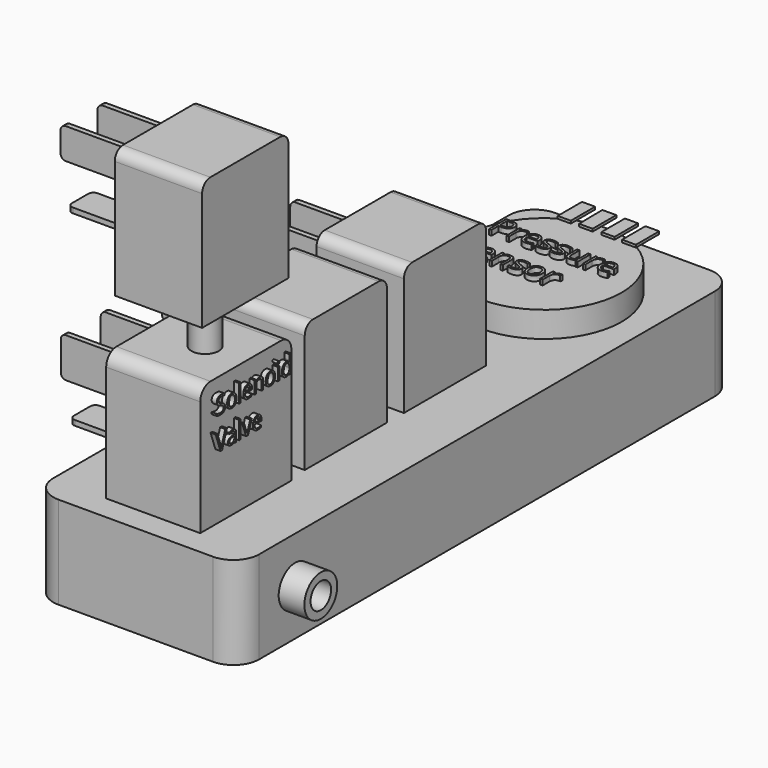
from build123d import *

# Parameters (mm, degrees)
F0_W          = 40.0781370699
F0_H          = 120.8194904029
F1_DEPTH      = 18
F2_R          = 15.0946600393
F3_DEPTH      = 5
F5_DEPTH      = 0.5
F7_DEPTH      = 0.5
F9_DEPTH      = 0.5
F10_TEXT_SIZE = 5.8368311741
F11_DEPTH     = 1
F12_R         = 4
F13_DEPTH     = 5
F15_D         = 5
F15_DEPTH     = 10
F15_TIP       = 1.5021515476
F17_DEPTH     = 0.5
F18_R         = 4
F19_DEPTH     = 5
F21_D         = 5
F21_DEPTH     = 10
F21_TIP       = 1.5021515476
F22_R         = 5
F23_R         = 5
F24_R         = 5
F25_R         = 5
F26_W         = 18.3048888575
F26_H         = 22.1605543047
F27_DEPTH     = 25
F28_R         = 2.5
F29_TEXT_SIZE = 4.6175733077
F30_DEPTH     = 1
F31_W         = 17
F31_H         = 20
F32_DEPTH     = 25
F33_R         = 2
F35_W         = 1
F35_H         = 7.7205877751
F35_W_2       = 6
F35_H_2       = 1
F36_DEPTH     = 15
F37_R         = 2.6676591168
F38_DEPTH     = 10
F39_W         = 17
F39_H         = 21
F40_DEPTH     = 25
F41_R         = 2
F42_W         = 1
F42_H         = 6
F42_W_2       = 6
F42_H_2       = 1
F43_DEPTH     = 15
F44_R         = 1


# Not quite as in the source:
# - Text() gives the source's letters only with a copy of the font that has no kerning and outlines rounded to 1/6400 em; it was checked with that copy


with BuildPart() as f1:
    # F0 (on Top) → F1 (new body)
    with BuildSketch(Plane.XY):
        with Locations((-11.1165624112, 8.9225042611)):
            Rectangle(F0_W, F0_H)
    extrude(amount=F1_DEPTH)

    # F2 (on face) → F3 (join)
    with BuildSketch(Plane.XY.offset(18)):
        with Locations((-10.9592955559, 47.6713515818)):
            Circle(F2_R)
    extrude(amount=F3_DEPTH)

    # F4 (on face) → F5 (join)
    with BuildSketch(Plane.XY.offset(23)):
        with BuildLine():
            Line((-14.5544850931, 66.3335174322), (-14.4999837088, 62.3448749864))
            ThreePointArc((-14.4999837088, 62.3448749864), (-13.1815212085, 62.6015382803), (-11.8454620242, 62.7399769568))
            Line((-11.8454620242, 62.7399769568), (-11.8454620242, 66.3335174322))
            Line((-11.8454620242, 66.3335174322), (-14.5544850931, 66.3335174322))
        make_face()
        with BuildLine():
            Line((-14.4999837088, 62.3448749864), (-14.4758609787, 60.5794712901))
            Line((-14.4758609787, 60.5794712901), (-11.8454620242, 60.5794712901))
            Line((-11.8454620242, 60.5794712901), (-11.8454620242, 62.7399769568))
            ThreePointArc((-11.8454620242, 62.7399769568), (-13.1815212085, 62.6015382803), (-14.4999837088, 62.3448749864))
        make_face()
    extrude(amount=F5_DEPTH)

    # F6 (on face) → F7 (join)
    with BuildSketch(Plane.XY.offset(23)):
        with BuildLine():
            Line((-18.6310531572, 60.5794712901), (-16.0875776783, 60.5794712901))
            Line((-16.0875776783, 60.5794712901), (-16.0875776783, 61.8681640471))
            ThreePointArc((-16.0875776783, 61.8681640471), (-17.3872429539, 61.3289594965), (-18.6310531572, 60.671078387))
            Line((-18.6310531572, 60.671078387), (-18.6310531572, 60.5794712901))
        make_face()
        with BuildLine():
            ThreePointArc((-18.6310531572, 60.671078387), (-17.3872429539, 61.3289594965), (-16.0875776783, 61.8681640471))
            Line((-16.0875776783, 61.8681640471), (-16.0875776783, 66.4905309677))
            Line((-16.0875776783, 66.4905309677), (-18.6310531572, 66.4905309677))
            Line((-18.6310531572, 66.4905309677), (-18.6310531572, 60.671078387))
        make_face()
    extrude(amount=F7_DEPTH)

    # F8 (on face) → F9 (join)
    with BuildSketch(Plane.XY.offset(23)):
        with BuildLine():
            Line((-10.1195760071, 66.2886723876), (-10.1195760071, 62.7426366226))
            ThreePointArc((-10.1195760071, 62.7426366226), (-8.8371052881, 62.6160854426), (-7.5701028109, 62.380604936))
            Line((-7.5701028109, 62.380604936), (-7.5701028109, 66.2886723876))
            Line((-7.5701028109, 66.2886723876), (-10.1195760071, 66.2886723876))
        make_face()
        with BuildLine():
            Line((-10.1195760071, 62.7426366226), (-10.1195760071, 60.5794712901))
            Line((-10.1195760071, 60.5794712901), (-7.5701028109, 60.5794712901))
            Line((-7.5701028109, 60.5794712901), (-7.5701028109, 62.380604936))
            ThreePointArc((-7.5701028109, 62.380604936), (-8.8371052881, 62.6160854426), (-10.1195760071, 62.7426366226))
        make_face()
    extrude(amount=F9_DEPTH)

    # F10 (on face) → F11 (join)
    with BuildSketch(Plane.XY.offset(23)):
        with Locations((-24.0541284715, 49.934240443)):
            Text('Pressure', F10_TEXT_SIZE, font='Open Sans', text_align=(TextAlign.LEFT, TextAlign.BOTTOM))
        with Locations((-24.0541284715, 41.9961500462)):
            Text('Sensor', F10_TEXT_SIZE, font='Open Sans', text_align=(TextAlign.LEFT, TextAlign.BOTTOM))
    extrude(amount=F11_DEPTH)

    # F12 (on face) → F13 (join)
    with BuildSketch(Plane(origin=(0, 69.3322494626, 0), x_dir=(-1, 0, 0), z_dir=(0, 1, 0))):
        with Locations((11.1165624112, 9)):
            Circle(F12_R)
    extrude(amount=F13_DEPTH)

    # F15
    with Locations(Plane(origin=(0, 74.3322494626, 0), x_dir=(-1, 0, 0), z_dir=(0, 1, 0))):
        with Locations((11.1165624112, 9)):
            Hole(F15_D / 2, depth=F15_DEPTH)
            with Locations((0, 0, -(F15_DEPTH + F15_TIP / 2))):  # 118° drill point
                Cone(0, F15_D / 2, F15_TIP, mode=Mode.SUBTRACT)

    # F16 (on face) → F17 (join)
    with BuildSketch(Plane.XY.offset(23)):
        with BuildLine():
            Line((-6.1028422788, 61.9634341197), (-6.1028422788, 60.5794712901))
            Line((-6.1028422788, 60.5794712901), (-3.4190774895, 60.5794712901))
            Line((-3.4190774895, 60.5794712901), (-3.4190774895, 60.7478141468))
            ThreePointArc((-3.4190774895, 60.7478141468), (-4.7312301998, 61.4212593496), (-6.1028422788, 61.9634341197))
        make_face()
        with BuildLine():
            Line((-6.1028422788, 66.256262362), (-6.1028422788, 61.9634341197))
            ThreePointArc((-6.1028422788, 61.9634341197), (-4.7312301998, 61.4212593496), (-3.4190774895, 60.7478141468))
            Line((-3.4190774895, 60.7478141468), (-3.4190774895, 66.256262362))
            Line((-3.4190774895, 66.256262362), (-6.1028422788, 66.256262362))
        make_face()
    extrude(amount=F17_DEPTH)

    # F18 (on face) → F19 (join)
    with BuildSketch(Plane.YZ.offset(8.9225061238)):
        with Locations((-37.7472043037, 9)):
            Circle(F18_R)
    extrude(amount=F19_DEPTH)

    # F21
    with Locations(Plane.YZ.offset(13.9225061238)):
        with Locations((-37.7472043037, 9)):
            Hole(F21_D / 2, depth=F21_DEPTH)
            with Locations((0, 0, -(F21_DEPTH + F21_TIP / 2))):  # 118° drill point
                Cone(0, F21_D / 2, F21_TIP, mode=Mode.SUBTRACT)

    # F22
    f22_edges = [f1.edges().sort_by_distance(p)[0] for p in [
        (8.922506, 69.332249, 9),
    ]]
    fillet(f22_edges, radius=F22_R)

    # F23
    f23_edges = [f1.edges().sort_by_distance(p)[0] for p in [
        (-31.155631, 69.332249, 9),
    ]]
    fillet(f23_edges, radius=F23_R)

    # F24
    f24_edges = [f1.edges().sort_by_distance(p)[0] for p in [
        (-31.155631, -51.487241, 9),
    ]]
    fillet(f24_edges, radius=F24_R)

    # F25
    f25_edges = [f1.edges().sort_by_distance(p)[0] for p in [
        (8.922506, -51.487241, 9),
    ]]
    fillet(f25_edges, radius=F25_R)

    # F26 (on face) → F27 (join)
    with BuildSketch(Plane.XY.offset(18)):
        with Locations((-11.564587825, -35.5752883479)):
            Rectangle(F26_W, F26_H)
    extrude(amount=F27_DEPTH)

    # F28
    f28_edges = [f1.edges().sort_by_distance(p)[0] for p in [
        (-11.564588, -46.655566, 43),
        (-11.564588, -24.495011, 43),
    ]]
    fillet(f28_edges, radius=F28_R)

    # F29 (on face) → F30 (join)
    with BuildSketch(Plane.YZ.offset(-2.4121433962)):
        with Locations((-44.1555655003, 37.1753472185)):
            Text('Solenoid', F29_TEXT_SIZE, font='Open Sans', text_align=(TextAlign.LEFT, TextAlign.BOTTOM))
        with Locations((-44.1555655003, 30.8954475201)):
            Text('Valve', F29_TEXT_SIZE, font='Open Sans', text_align=(TextAlign.LEFT, TextAlign.BOTTOM))
    extrude(amount=F30_DEPTH)

    # F31 (on face) → F32 (join)
    with BuildSketch(Plane.XY.offset(18)):
        with Locations((-11.4914905614, -10.5143212713)):
            Rectangle(F31_W, F31_H)
        with Locations((-11.4474429283, 13.5548580438)):
            Rectangle(F31_W, F31_H)
    extrude(amount=F32_DEPTH)

    # F33
    f33_edges = [f1.edges().sort_by_distance(p)[0] for p in [
        (-11.491491, -0.514321, 43),
        (-11.491491, -20.514321, 43),
        (-11.447443, 3.554858, 43),
        (-11.447443, 23.554858, 43),
    ]]
    fillet(f33_edges, radius=F33_R)

    # F35 (on offset) → F36 (join)
    with BuildSketch(Plane(origin=(-19.9474429283, 0, 0), x_dir=(0, -1, 0), z_dir=(-1, 0, 0))):
        with Locations((-8.8547184952, 35.0220622495)):
            Rectangle(F35_W, F35_H)
        with Locations((-16.4049044251, 35.12294963)):
            Rectangle(F35_W, F35_H)
        with Locations((14.7996973246, 35.016624257)):
            Rectangle(F35_W, F35_H)
        with Locations((6.7987809889, 35.0161008537)):
            Rectangle(F35_W, F35_H)
        with Locations((29.6944491565, 35.014366731)):
            Rectangle(F35_W, F35_H)
        with Locations((39.4039042294, 35.0501220673)):
            Rectangle(F35_W, F35_H)
        with Locations((34.7302383482, 23.0127320737)):
            Rectangle(F35_W_2, F35_H_2)
        with Locations((10.6482356787, 23.0187382549)):
            Rectangle(F35_W_2, F35_H_2)
        with Locations((-12.8180906177, 22.5305911154)):
            Rectangle(F35_W_2, F35_H_2)
    extrude(amount=F36_DEPTH)

    # F37 (on face) → F38 (join)
    with BuildSketch(Plane.XY.offset(43)):
        with Locations((-10.3327590041, -35.5752883479)):
            Circle(F37_R)
    extrude(amount=F38_DEPTH)

    # F39 (on face) → F40 (join)
    with BuildSketch(Plane.XY.offset(53)):
        with Locations((-10.8921907376, -35.7271866826)):
            Rectangle(F39_W, F39_H)
    extrude(amount=F40_DEPTH)

    # F41
    f41_edges = [f1.edges().sort_by_distance(p)[0] for p in [
        (-10.892191, -25.227187, 78),
        (-10.892191, -46.227187, 78),
    ]]
    fillet(f41_edges, radius=F41_R)

    # F42 (on face) → F43 (join)
    with BuildSketch(Plane(origin=(-19.3921907376, 0, 0), x_dir=(0, -1, 0), z_dir=(-1, 0, 0))):
        with Locations((40.155082099, 72.2279399633)):
            Rectangle(F42_W, F42_H)
        with Locations((31.1569842398, 72.0812468529)):
            Rectangle(F42_W, F42_H)
        with Locations((35.9090543091, 60.0747940242)):
            Rectangle(F42_W_2, F42_H_2)
    extrude(amount=F43_DEPTH)

    # F44
    f44_edges = [f1.edges().sort_by_distance(p)[0] for p in [
        (-34.947443, 9.818091, 22.530591),
        (-34.947443, 15.818091, 22.530591),
        (-34.947443, 16.404904, 31.262656),
        (-34.947443, 8.854718, 31.161768),
        (-34.947443, 8.854718, 38.882356),
        (-34.947443, 16.404904, 38.983244),
        (-34.947443, -6.798781, 38.876395),
        (-34.947443, -6.798781, 31.155807),
        (-34.947443, -14.799697, 31.15633),
        (-34.947443, -14.799697, 38.876918),
        (-34.947443, -13.648236, 23.018738),
        (-34.947443, -7.648236, 23.018738),
        (-34.947443, -39.403904, 31.189828),
        (-34.947443, -29.694449, 31.154073),
        (-34.947443, -29.694449, 38.874661),
        (-34.947443, -39.403904, 38.910416),
        (-34.947443, -37.730238, 23.012732),
        (-34.947443, -31.730238, 23.012732),
        (-34.392191, -38.909054, 60.074794),
        (-34.392191, -32.909054, 60.074794),
        (-34.392191, -31.156984, 75.081247),
        (-34.392191, -31.156984, 69.081247),
        (-34.392191, -40.155082, 69.22794),
        (-34.392191, -40.155082, 75.22794),
    ]]
    fillet(f44_edges, radius=F44_R)


solid = f1.part
